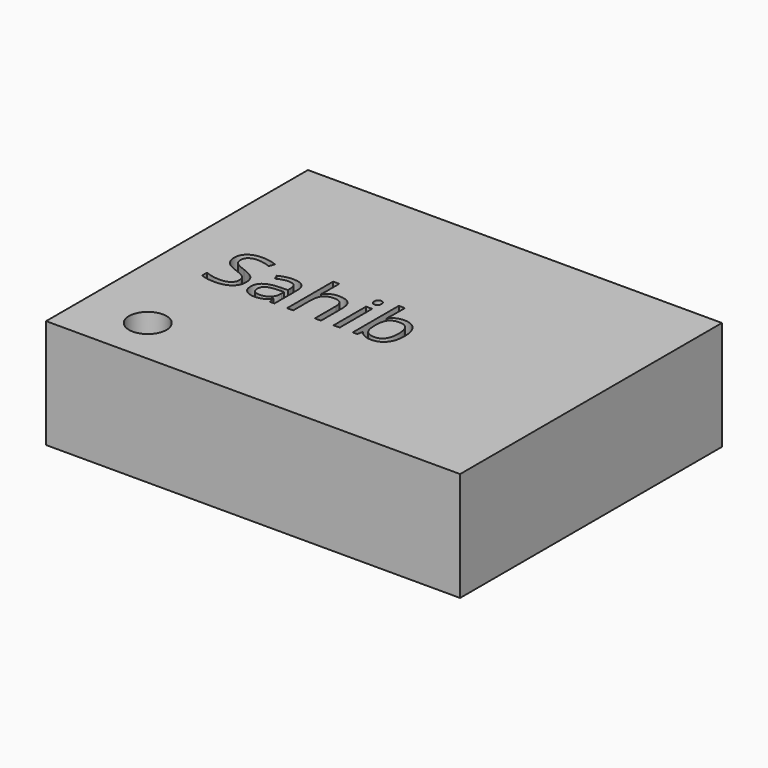
from build123d import *

# Parameters (mm, degrees)
F2_W         = 96.3943435967
F2_H         = 76.2
F2_R         = 4.3698755439
F3_DEPTH     = 25.4
F0_TEXT_SIZE = 17.6388888889
F4_DEPTH     = 25.4


# Not quite as in the source:
# - Text() gives the source's letters only with a copy of the font that has no kerning and outlines rounded to 1/6400 em; it was checked with that copy


with BuildPart() as f3:
    # F2 (on face) → F3 (new body)
    with BuildSketch(Plane.XY):
        with Locations((11.9711337611, 21.5156232007)):
            Rectangle(F2_W, F2_H)
        with Locations((-21.3377531618, -5.6041134521)):
            Circle(F2_R, mode=Mode.SUBTRACT)
    extrude(amount=F3_DEPTH)

    # F0 (on Top) → F4 (cut)
    with BuildSketch(Plane.XY):
        with Locations((-26.2167728813, 14.7797156453)):
            Text('Sahib', F0_TEXT_SIZE, font='Open Sans', text_align=(TextAlign.LEFT, TextAlign.BOTTOM))
    extrude(amount=F4_DEPTH, mode=Mode.SUBTRACT)


solid = f3.part
